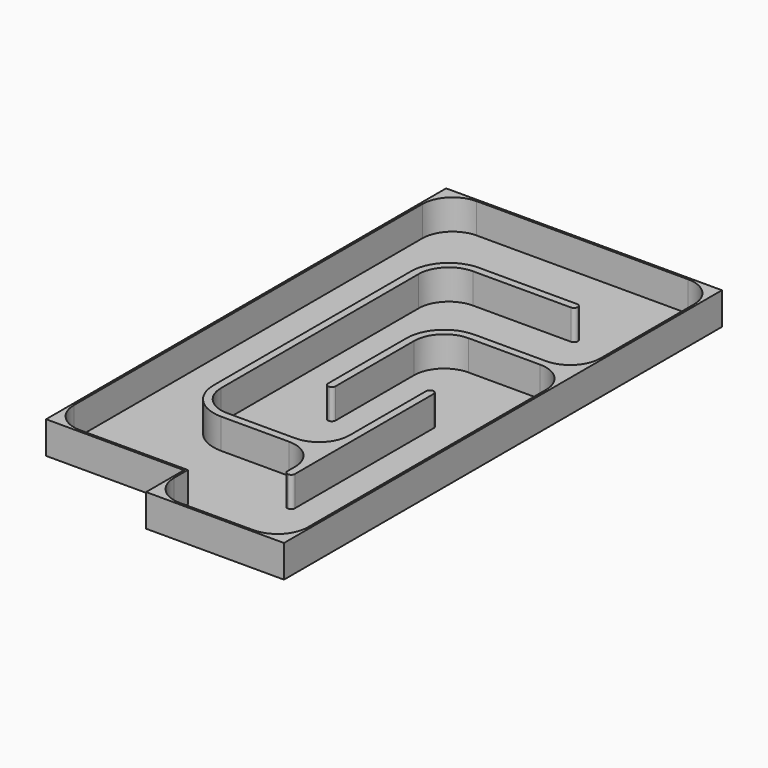
from build123d import *

# Parameters (mm, degrees)
F6_DEPTH      = 200
F6_DEPTH_BACK = 14
F7_T          = -14
F12_W         = 50
F12_H         = 200
F13_W         = 50
F13_H         = 200
F14_W         = 50
F14_H         = 200
F19_R         = 200
F19_2_R       = 200
F20_R         = 250
F20_2_R       = 250
F21_R         = 24.99999
F21_2_R       = 24.99999


# Not quite as in the source:
# - a fillet or chamfer is up to 0.001 mm smaller than in the source, because OpenCascade refuses the exact size


with BuildPart() as f6:
    # F5 (on Top) → F6 (new body, two sides)
    with BuildSketch(Plane.XY) as f6_sk:
        Polygon((914, 1814), (-914, 1814), (-914, -1500), (0, -1500), (0, -1814), (914, -1814), align=None)
    extrude(amount=F6_DEPTH)
    extrude(f6_sk.sketch, amount=-F6_DEPTH_BACK)

    # F7
    f7_openings = [f6.faces().sort_by_distance(p)[0] for p in [
        (20.670988, 74.949294, 200),
    ]]
    offset(amount=F7_T, openings=f7_openings, kind=Kind.INTERSECTION)

    # F17: sweep along a path in F8
    with BuildLine(Plane.XY) as f17_path:
        Line((0, -300), (0, 600))
        Line((0, 600), (900, 600))
    # F14 (on plane+point) → F17 (sweep)
    with BuildSketch(Plane.XZ.offset(300)):
        with Locations((0, 100)):
            Rectangle(F14_W, F14_H)
    sweep(path=f17_path.line, transition=Transition.RIGHT)

    # F19
    f19_edges = [f6.edges().sort_by_distance(p)[0] for p in [
        (25, 575, 100),
        (900, 575, 100),
        (900, 625, 100),
        (14, -1800, 100),
        (900, -1800, 100),
        (-900, -1486, 100),
        (-900, 1800, 100),
        (900, 1800, 100),
    ]]
    fillet(f19_edges, radius=F19_R)

    # F20
    f20_edges = [f6.edges().sort_by_distance(p)[0] for p in [
        (-25, 625, 100),
    ]]
    fillet(f20_edges, radius=F20_R)

    # F21 (radius 25 in the source; OpenCascade refuses exactly that, so slightly less here)
    f21_edges = [f6.edges().sort_by_distance(p)[0] for p in [
        (25, -300, 100),
        (-25, -300, 100),
    ]]
    fillet(f21_edges, radius=F21_R)


with BuildPart() as f15:
    # F15: sweep along a path in F8
    with BuildLine(Plane.XY) as f15_path:
        Line((450, 1200), (-450, 1200))
        Line((-450, 1200), (-450, -886))
        Line((-450, -886), (450, -886))
    # F12 (on plane+point) → F15 (sweep)
    with BuildSketch(Plane.YZ.offset(450)):
        with Locations((1200, 100)):
            Rectangle(F12_W, F12_H)
    sweep(path=f15_path.line, transition=Transition.RIGHT)

    # F16: sweep along a path in F8
    with BuildLine(Plane.XY) as f16_path:
        Line((450, -1200), (450, 0))
    # F13 (on plane+point) → F16 (sweep)
    with BuildSketch(Plane.XZ.offset(1200)):
        with Locations((450, 100)):
            Rectangle(F13_W, F13_H)
    sweep(path=f16_path.line)

    # F18: union 

    # F19#2
    f19_2_edges = [f15.edges().sort_by_distance(p)[0] for p in [
        (425, -861, 100),
        (-425, -861, 100),
        (-425, 1175, 100),
        (425, -911, 100),
    ]]
    fillet(f19_2_edges, radius=F19_2_R)

    # F20#2
    f20_2_edges = [f15.edges().sort_by_distance(p)[0] for p in [
        (-475, 1225, 100),
        (-475, -911, 100),
    ]]
    fillet(f20_2_edges, radius=F20_2_R)

    # F21#2 (radius 25 in the source; OpenCascade refuses exactly that, so slightly less here)
    f21_2_edges = [f15.edges().sort_by_distance(p)[0] for p in [
        (450, 1225, 100),
        (450, 1175, 100),
        (425, 0, 100),
        (475, 0, 100),
        (425, -1200, 100),
        (475, -1200, 100),
    ]]
    fillet(f21_2_edges, radius=F21_2_R)


solid = Compound([f6.part, f15.part])
